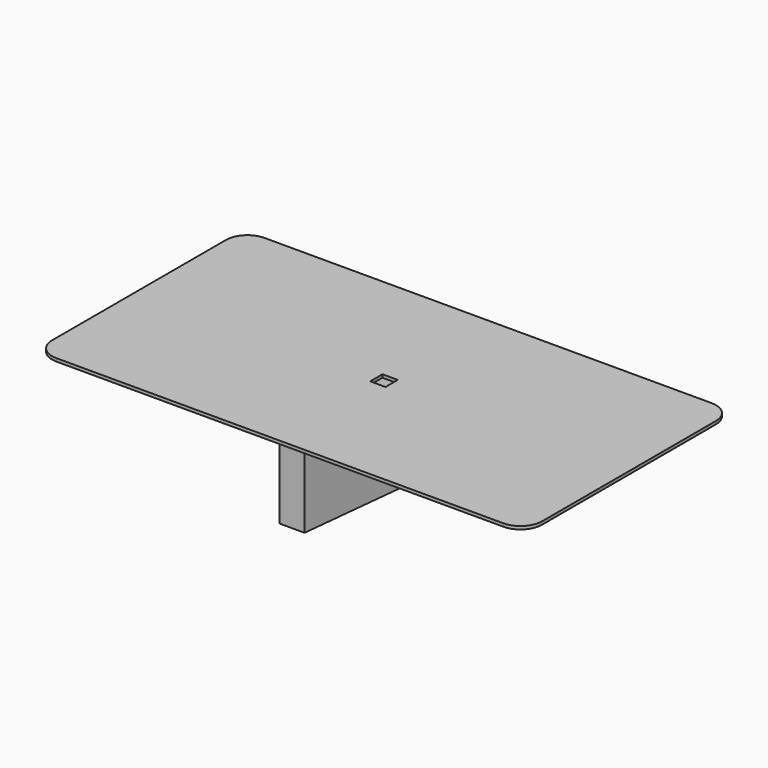
from build123d import *

# Parameters (mm, degrees)
F0_R     = 8
F1_DEPTH = 1
F4_W     = 5
F4_H     = 5
F5_DEPTH = 25
F6_DEPTH = 26.197


with BuildPart() as f1:
    # F0 (on Top) → F1 (new body)
    with BuildSketch(Plane.XY):
        with BuildLine():
            Line((-73, -42.5), (73, -42.5))
            ThreePointArc((73, -42.5), (77.9497474683, -40.4497474683), (80, -35.5))
            Line((80, -35.5), (80, 35.5))
            ThreePointArc((80, 35.5), (77.9497474683, 40.4497474683), (73, 42.5))
            Line((73, 42.5), (-73, 42.5))
            ThreePointArc((-73, 42.5), (-77.9497474683, 40.4497474683), (-80, 35.5))
            Line((-80, 35.5), (-80, -35.5))
            ThreePointArc((-80, -35.5), (-77.9497474683, -40.4497474683), (-73, -42.5))
        make_face()
        Circle(F0_R, mode=Mode.SUBTRACT)
        Circle(F0_R)
    extrude(amount=F1_DEPTH)

    # F4 (on face) → F5 (cut)
    with BuildSketch(Plane(origin=(0, 0, 0), x_dir=(1, 0, 0), z_dir=(0, 0, -1))):
        Rectangle(F4_W, F4_H)
    extrude(amount=-F5_DEPTH, mode=Mode.SUBTRACT)

    # F3 (on face) → F6 (join)
    with BuildSketch(Plane(origin=(0, 0, 0), x_dir=(1, 0, 0), z_dir=(0, 0, -1))):
        with BuildLine():
            ThreePointArc((-7.8251753865, 1.6633190224), (0, 8), (7.8251753865, 1.6633190224))
            Line((7.8251753865, 1.6633190224), (5.3723529412, 25))
            Line((5.3723529412, 25), (-5.3723529412, 25))
            Line((-5.3723529412, 25), (-7.8251753865, 1.6633190224))
        make_face()
        with BuildLine():
            Line((6.4233442804, -15), (7.8251605833, -1.6633886632))
            ThreePointArc((7.8251605833, -1.6633886632), (-3.55984e-05, -7.9999999999), (-7.8251753865, -1.6633190224))
            Line((-7.8251753865, -1.6633190224), (-6.4234117647, -15))
            Line((-6.4234117647, -15), (3.0757090009, -15))
            Line((3.0757090009, -15), (6.4233442804, -15))
        make_face()
        Polygon((-5.3723529412, 25), (5.3723529412, 25), (4.0585294118, 37.5), (-4.0585294118, 37.5), align=None)
        Polygon((4.0583607009, -37.5), (6.4233442804, -15), (3.0757090009, -15), (-6.4234117647, -15), (-4.0585294118, -37.5), align=None)
    extrude(amount=F6_DEPTH)


solid = f1.part
